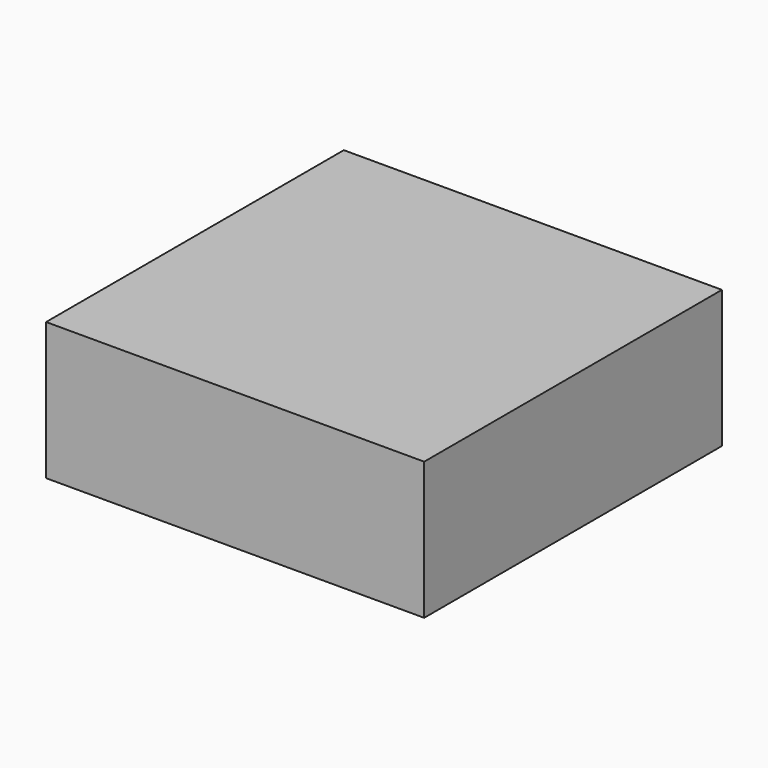
from build123d import *

# Parameters (mm, degrees)
F0_W     = 69.8630958796
F0_H     = 137.5265717506
F2_DEPTH = 50.8


# Not quite as in the source:
# - the program builds the solid bodies; features that only make, move or delete a surface that nothing else refers to are left out


with BuildPart() as f2:
    # F0 (on Top) → F2 (new body)
    with BuildSketch(Plane.XY):
        with Locations((-34.9315479398, 0)):
            Rectangle(F0_W, F0_H)
        with Locations((34.9315479398, 0)):
            Rectangle(F0_W, F0_H)
    extrude(amount=-F2_DEPTH)


solid = f2.part
